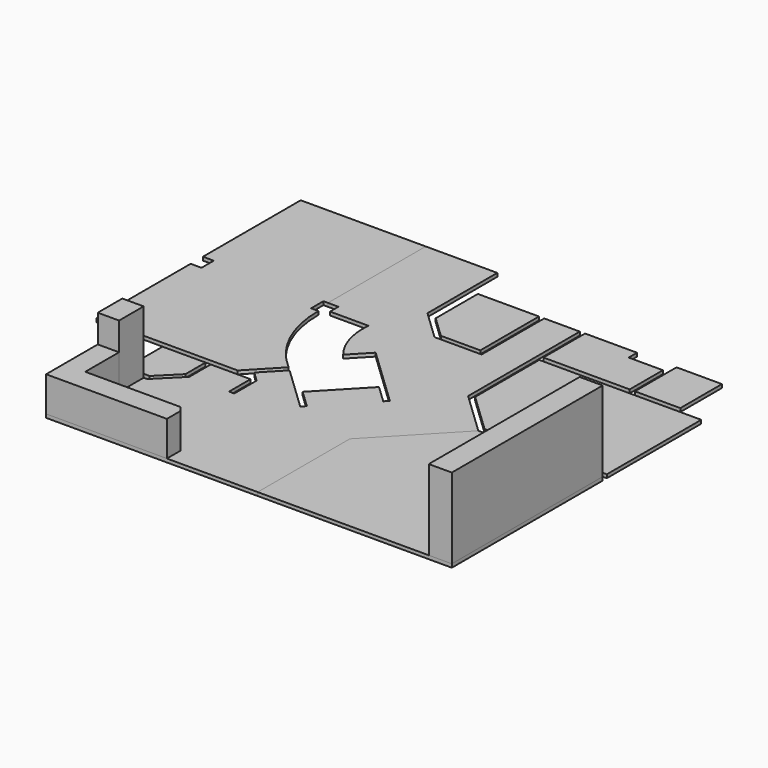
from build123d import *

# Parameters (mm, degrees)
F1_DEPTH  = 100
F0_W      = 660
F0_H      = 5400
F2_DEPTH  = 100
F3_DEPTH  = 100
F4_DEPTH  = 100
F5_DEPTH  = 100
F0_W_2    = 1300
F0_H_2    = 1490
F6_DEPTH  = 100
F7_DEPTH  = 100
F0_W_3    = 610
F0_H_3    = 880
F8_DEPTH  = 100
F9_DEPTH  = 1000
F10_DEPTH = 1800
F11_DEPTH = 2300


# Not quite as in the source:
# - a feature names something its author has since deleted; it is built from what else it names


with BuildPart() as f1:
    # F0 (on Top) → F1 (new body)
    with BuildSketch(Plane.XY):
        with BuildLine():
            Line((-2600, 488.0131584643), (-2600, 0))
            Line((-2600, 0), (0, 0))
            Line((0, 0), (0, 3300))
            Line((0, 3300), (2000, 5400))
            Line((2000, 5400), (770, 6571.4285714286))
            Line((770, 6571.4285714286), (770, 10570))
            Line((770, 10570), (-250, 10570))
            Line((-250, 10570), (-250, 8330))
            Line((-250, 8330), (-1600, 8330))
            Line((-1600, 8330), (-2447.2413793103, 9136.8965517241))
            Line((-2447.2413793103, 9136.8965517241), (-2447.2413793103, 11636.8965517241))
            Line((-2447.2413793103, 11636.8965517241), (-4497.2413793103, 11636.8965517241))
            Line((-4497.2413793103, 11636.8965517241), (-4497.2413793103, 8136.8965517241))
            Line((-4497.2413793103, 8136.8965517241), (-4197.2413793103, 8136.8965517241))
            Line((-4197.2413793103, 8136.8965517241), (-4197.2413793103, 7836.8965517241))
            Line((-4197.2413793103, 7836.8965517241), (-3097.2413793103, 7836.8965517241))
            ThreePointArc((-3097.2413793103, 7836.8965517241), (-3021.9650759345, 7071.0659908147), (-2663.1034482759, 6390.3448275862))
            Line((-2663.1034482759, 6390.3448275862), (-2157.5862068966, 6921.1379310345))
            Line((-2157.5862068966, 6921.1379310345), (-448.6206896552, 5293.5517241379))
            Line((-448.6206896552, 5293.5517241379), (-552.0689655172, 5184.9310344828))
            Line((-552.0689655172, 5184.9310344828), (-1058.9655172414, 5667.6896551724))
            Line((-1058.9655172414, 5667.6896551724), (-2247.2413793103, 4420))
            Line((-2247.2413793103, 4420), (-1740.3448275862, 3937.2413793103))
            Line((-1740.3448275862, 3937.2413793103), (-1843.7931034483, 3828.6206896552))
            Line((-1843.7931034483, 3828.6206896552), (-3125.5172413793, 5049.3103448276))
            Line((-3125.5172413793, 5049.3103448276), (-3675.4618885563, 4471.8684652917))
            Line((-3675.4618885563, 4471.8684652917), (-3390, 4200))
            Line((-3390, 4200), (-3390, 3400))
            Line((-3390, 3400), (-3540, 3400))
            Line((-3540, 3400), (-3540, 4170))
            Line((-3540, 4170), (-4680, 4170))
            Line((-4680, 4170), (-4680, 3400))
            Line((-4680, 3400), (-4821.4213562373, 3258.5786437627))
            Line((-4821.4213562373, 3258.5786437627), (-5350, 2730))
            Line((-5350, 2730), (-5450, 2730))
            Line((-5450, 2730), (-5450, 1850))
            Line((-5450, 1850), (-5450, 640))
            Line((-5450, 640), (-2730, 640))
            Line((-2730, 640), (-2600, 488.0131584643))
        make_face()
    extrude(amount=-F1_DEPTH)

    # F0 (on Top) → F8 (join)
    with BuildSketch(Plane.XY):
        Polygon((-6060, 0), (-2600, 0), (-2600, 488.0131584643), (-2730, 640), (-5450, 640), (-5450, 1850), (-6060, 1850), align=None)
        with Locations((-5755, 2290)):
            Rectangle(F0_W_3, F0_H_3)
    extrude(amount=-F8_DEPTH)


with BuildPart() as f1b:
    # F0 (on Top) → F1, piece 2 (new body)
    with BuildSketch(Plane.XY):
        Polygon((-6060, 4170), (-6060, 2880), (-5400, 2880), (-4921.4213562373, 3358.5786437627), (-4830, 3450), (-4830, 4170), (-5900, 4170), align=None)
    extrude(amount=-F1_DEPTH)


with BuildPart() as f2:
    # F0 (on Top) → F2 (new body)
    with BuildSketch(Plane.XY):
        Polygon((0, 3300), (0, 0), (4900, 0), (4900, 5400), (2000, 5400), align=None)
        with Locations((5230, 2700)):
            Rectangle(F0_W, F0_H)
    extrude(amount=-F2_DEPTH)


with BuildPart() as f3:
    # F0 (on Top) → F3 (new body)
    with BuildSketch(Plane.XY):
        with BuildLine():
            Line((-8077.2413793103, 4320), (-6060, 4320))
            Line((-6060, 4320), (-4027.2413793103, 4320))
            Line((-4027.2413793103, 4320), (-3234.1379310345, 5152.7586206897))
            ThreePointArc((-3234.1379310345, 5152.7586206897), (-4109.5423503056, 6292.8272342142), (-4417.2413793103, 7696.8965517241))
            Line((-4417.2413793103, 7696.8965517241), (-4627.2413793103, 7696.8965517241))
            Line((-4627.2413793103, 7696.8965517241), (-4627.2413793103, 8136.8965517241))
            Line((-4627.2413793103, 8136.8965517241), (-4497.2413793103, 8136.8965517241))
            Line((-4497.2413793103, 8136.8965517241), (-4497.2413793103, 11636.8965517241))
            Line((-4497.2413793103, 11636.8965517241), (-8077.2413793103, 11636.8965517241))
            Line((-8077.2413793103, 11636.8965517241), (-8077.2413793103, 8136.8965517241))
            Line((-8077.2413793103, 8136.8965517241), (-7767.2413793103, 8136.8965517241))
            Line((-7767.2413793103, 8136.8965517241), (-7767.2413793103, 7696.8965517241))
            Line((-7767.2413793103, 7696.8965517241), (-8077.2413793103, 7696.8965517241))
            Line((-8077.2413793103, 7696.8965517241), (-8077.2413793103, 4320))
        make_face()
    extrude(amount=-F3_DEPTH)


with BuildPart() as f4:
    # F0 (on Top) → F4 (new body)
    with BuildSketch(Plane.XY):
        Polygon((-400, 8470), (-400, 10570), (-2150, 10570), (-2150, 9060.9523809524), (-1529.5, 8470), align=None)
    extrude(amount=-F4_DEPTH)


with BuildPart() as f5:
    # F0 (on Top) → F5 (new body)
    with BuildSketch(Plane.XY):
        Polygon((4900, 5550), (5560, 5550), (5560, 8930), (920, 8930), (920, 6635.7142857143), (2060, 5550), align=None)
    extrude(amount=-F5_DEPTH)


with BuildPart() as f6:
    # F0 (on Top) → F6 (new body)
    with BuildSketch(Plane.XY):
        with Locations((4190, 9825)):
            Rectangle(F0_W_2, F0_H_2)
    extrude(amount=-F6_DEPTH)


with BuildPart() as f7:
    # F0 (on Top) → F7 (new body)
    with BuildSketch(Plane.XY):
        Polygon((2410, 10570), (920, 10570), (920, 9080), (3390, 9080), (3390, 10270), (2410, 10270), align=None)
    extrude(amount=-F7_DEPTH)


with BuildPart() as f9:
    # F0 (on Top) → F9 (new body)
    with BuildSketch(Plane.XY):
        Polygon((-6060, 0), (-2600, 0), (-2600, 488.0131584643), (-2730, 640), (-5450, 640), (-5450, 1850), (-6060, 1850), align=None)
    extrude(amount=F9_DEPTH)


with BuildPart() as f10:
    # F0 (on Top) → F10 (new body)
    with BuildSketch(Plane.XY):
        with Locations((-5755, 2290)):
            Rectangle(F0_W_3, F0_H_3)
    extrude(amount=F10_DEPTH)


with BuildPart() as f11:
    # F0 (on Top) → F11 (new body)
    with BuildSketch(Plane.XY):
        with Locations((5230, 2700)):
            Rectangle(F0_W, F0_H)
    extrude(amount=F11_DEPTH)


solid = Compound([f1.part, f1b.part, f2.part, f3.part, f4.part, f5.part, f6.part, f7.part, f9.part, f10.part, f11.part])
